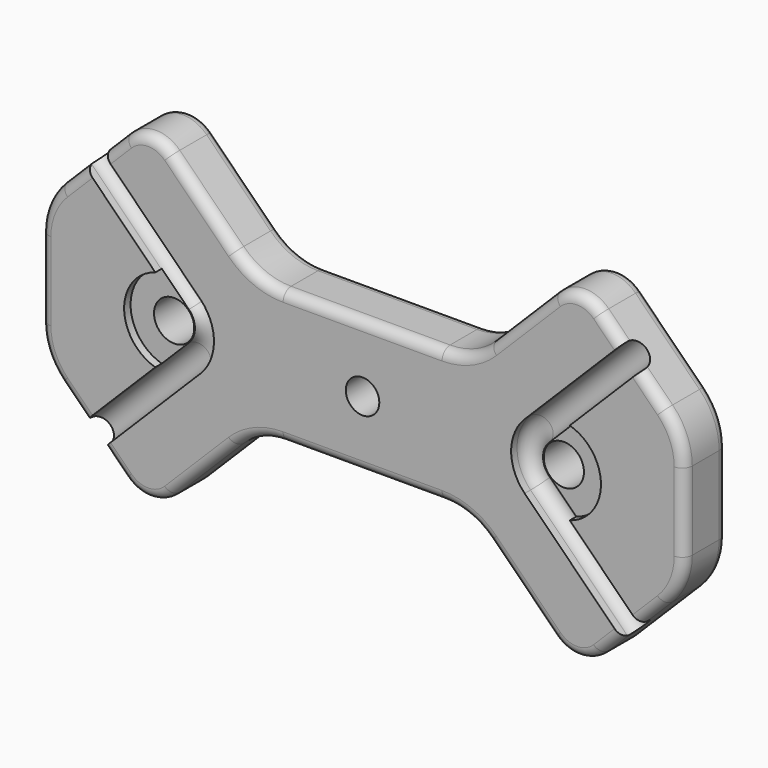
from build123d import *

# Parameters (mm, degrees)
F1_DEPTH  = 8
F4_R      = 6.5
F5_DEPTH  = 1.2
F6_R      = 3
F7_DEPTH  = 38
F9_R      = 2.5
F10_DEPTH = 22
F11_R     = 1.5


# Not quite as in the source:
# - a feature names something its author has since deleted; it is built from what else it names


with BuildPart() as f1:
    # F0 (on Front) → F1 (new body)
    with BuildSketch(Plane.XZ):
        with BuildLine():
            ThreePointArc((24.1920310217, -4.8790367902), (22.1710678119, 0), (24.1920310217, 4.8790367902))
            Line((24.1920310217, 4.8790367902), (38.6564971157, 19.3435028843))
            Line((38.6564971157, 19.3435028843), (35.5355339059, 22.4644660941))
            ThreePointArc((35.5355339059, 22.4644660941), (32, 23.9289321881), (28.4644660941, 22.4644660941))
            Line((28.4644660941, 22.4644660941), (18.9289321881, 12.9289321881))
            ThreePointArc((18.9289321881, 12.9289321881), (15.6846986999, 10.7612046749), (11.8578643763, 10))
            Line((11.8578643763, 10), (0, 10))
            Line((0, 10), (0, 0))
            Line((0, 0), (0, -10))
            Line((0, -10), (11.8578643763, -10))
            ThreePointArc((11.8578643763, -10), (15.6846986999, -10.7612046749), (18.9289321881, -12.9289321881))
            Line((18.9289321881, -12.9289321881), (28.4644660941, -22.4644660941))
            ThreePointArc((28.4644660941, -22.4644660941), (32, -23.9289321881), (35.5355339059, -22.4644660941))
            Line((35.5355339059, -22.4644660941), (38.6564971157, -19.3435028843))
            Line((38.6564971157, -19.3435028843), (24.1920310217, -4.8790367902))
        make_face()
        with BuildLine():
            Line((38.6564971157, 19.3435028843), (24.1920310217, 4.8790367902))
            ThreePointArc((24.1920310217, 4.8790367902), (22.1710678119, 0), (24.1920310217, -4.8790367902))
            Line((24.1920310217, -4.8790367902), (38.6564971157, -19.3435028843))
            Line((38.6564971157, -19.3435028843), (41.3435028843, -16.6564971157))
            Line((41.3435028843, -16.6564971157), (30.9188387655, -6.231832997))
            ThreePointArc((30.9188387655, -6.231832997), (22.5710678119, 0), (30.9188387655, 6.231832997))
            Line((30.9188387655, 6.231832997), (41.3435028843, 16.6564971157))
            Line((41.3435028843, 16.6564971157), (38.6564971157, 19.3435028843))
        make_face()
        with BuildLine():
            Line((45.0710678119, 12.9289321881), (41.3435028843, 16.6564971157))
            Line((41.3435028843, 16.6564971157), (30.9188387655, 6.231832997))
            ThreePointArc((30.9188387655, 6.231832997), (34.2797390051, 3.8884115524), (35.5710678119, 0))
            ThreePointArc((35.5710678119, 0), (34.2797390051, -3.8884115524), (30.9188387655, -6.231832997))
            Line((30.9188387655, -6.231832997), (41.3435028843, -16.6564971157))
            Line((41.3435028843, -16.6564971157), (45.0710678119, -12.9289321881))
            ThreePointArc((45.0710678119, -12.9289321881), (47.2387953251, -9.6846986999), (48, -5.8578643763))
            Line((48, -5.8578643763), (48, 5.8578643763))
            ThreePointArc((48, 5.8578643763), (47.2387953251, 9.6846986999), (45.0710678119, 12.9289321881))
        make_face()
        with BuildLine():
            ThreePointArc((35.5710678119, 0), (34.2797390051, 3.8884115524), (30.9188387655, 6.231832997))
            Line((30.9188387655, 6.231832997), (26.8790367902, 2.1920310217))
            ThreePointArc((26.8790367902, 2.1920310217), (25.9710678119, 0), (26.8790367902, -2.1920310217))
            Line((26.8790367902, -2.1920310217), (30.9188387655, -6.231832997))
            ThreePointArc((30.9188387655, -6.231832997), (34.2797390051, -3.8884115524), (35.5710678119, 0))
        make_face()
        with BuildLine():
            Line((26.8790367902, 2.1920310217), (30.9188387655, 6.231832997))
            ThreePointArc((30.9188387655, 6.231832997), (22.5710678119, 0), (30.9188387655, -6.231832997))
            Line((30.9188387655, -6.231832997), (26.8790367902, -2.1920310217))
            ThreePointArc((26.8790367902, -2.1920310217), (25.9710678119, 0), (26.8790367902, 2.1920310217))
        make_face()
    extrude(amount=-F1_DEPTH)

    # F3: sweep along a path in F0
    with BuildLine(Plane.XZ) as f3_path:
        Line((144.8327134998, 125.5197192683), (24.1920310217, 4.8790367902))
        ThreePointArc((24.1920310217, 4.8790367902), (22.1710678119, 0), (24.1920310217, -4.8790367902))
        Line((24.1920310217, -4.8790367902), (136.4443398617, -117.1313456302))
    # F2 (on face) → F3 (sweep, cut)
    with BuildSketch(Plane(origin=(29, 0, 29), x_dir=(0.7071067812, 0, -0.7071067812), z_dir=(0.7071067812, 0, 0.7071067812))):
        with BuildLine():
            Line((13.6563491861, 0), (17.4563491861, 0))
            Line((17.4563491861, 0), (17.4563491861, 1.0999976279))
            ThreePointArc((17.4563491861, 1.0999976279), (15.5563503722, 3), (13.6563491861, 1.1))
            Line((13.6563491861, 1.1), (13.6563491861, 0))
        make_face()
    sweep(path=f3_path.line, mode=Mode.SUBTRACT)

    # F4 (on face) → F5 (cut)
    with BuildSketch(Plane.XZ):
        with Locations((29.0710678119, 0)):
            Circle(F4_R)
    extrude(amount=-F5_DEPTH, mode=Mode.SUBTRACT)

    # F6 (on face) → F7 (cut)
    with BuildSketch(Plane.XZ):
        with Locations((29.0710678119, 0)):
            Circle(F6_R)
    extrude(amount=-F7_DEPTH, mode=Mode.SUBTRACT)

    # F8: F1 across plane


with BuildPart() as f1_1:
    add(f1.part)
    add(f1.part.mirror(Plane.YZ))

    # F9 (on face) → F10 (cut)
    with BuildSketch(Plane.XZ):
        Circle(F9_R)
    extrude(amount=-F10_DEPTH, mode=Mode.SUBTRACT)

    # F11
    f11_edges = [f1_1.edges().sort_by_distance(p)[0] for p in [
        (47.238795, 0, -9.684699),
        (23.696699, 0, 17.696699),
        (-48, 0, 0),
        (0, 0, -10),
        (0, 8, -10),
        (32, 0, 23.928932),
        (32, 8, 23.928932),
        (43.207285, 0, 14.792715),
        (37.096016, 0, 20.903984),
        (40.303301, 8, 17.696699),
        (23.696699, 8, 17.696699),
        (15.684699, 0, 10.761205),
        (37.096016, 0, -20.903984),
        (0, 0, 10),
        (32, 0, -23.928932),
        (-15.684699, 0, 10.761205),
        (23.696699, 0, -17.696699),
        (-23.696699, 0, 17.696699),
        (15.684699, 0, -10.761205),
        (-32, 0, 23.928932),
        (-37.096016, 0, 20.903984),
        (-15.684699, 0, -10.761205),
        (-23.696699, 0, -17.696699),
        (-32, 0, -23.928932),
        (-37.096016, 0, -20.903984),
        (47.238795, 8, 9.684699),
        (15.684699, 8, 10.761205),
        (48, 8, 0),
        (0, 8, 10),
        (47.238795, 8, -9.684699),
        (-15.684699, 8, 10.761205),
        (40.303301, 8, -17.696699),
        (-23.696699, 8, 17.696699),
        (32, 8, -23.928932),
        (-32, 8, 23.928932),
        (23.696699, 8, -17.696699),
        (-40.303301, 8, 17.696699),
        (15.684699, 8, -10.761205),
        (-47.238795, 8, 9.684699),
        (-48, 8, 0),
        (-15.684699, 8, -10.761205),
        (-47.238795, 8, -9.684699),
        (-23.696699, 8, -17.696699),
        (-40.303301, 8, -17.696699),
        (-32, 8, -23.928932),
        (47.238795, 0, 9.684699),
        (43.207285, 0, -14.792715),
        (48, 0, 0),
        (-43.207285, 0, 14.792715),
        (-43.207285, 0, -14.792715),
        (-47.238795, 0, 9.684699),
        (-47.238795, 0, -9.684699),
    ]]
    fillet(f11_edges, radius=F11_R)


solid = f1_1.part
